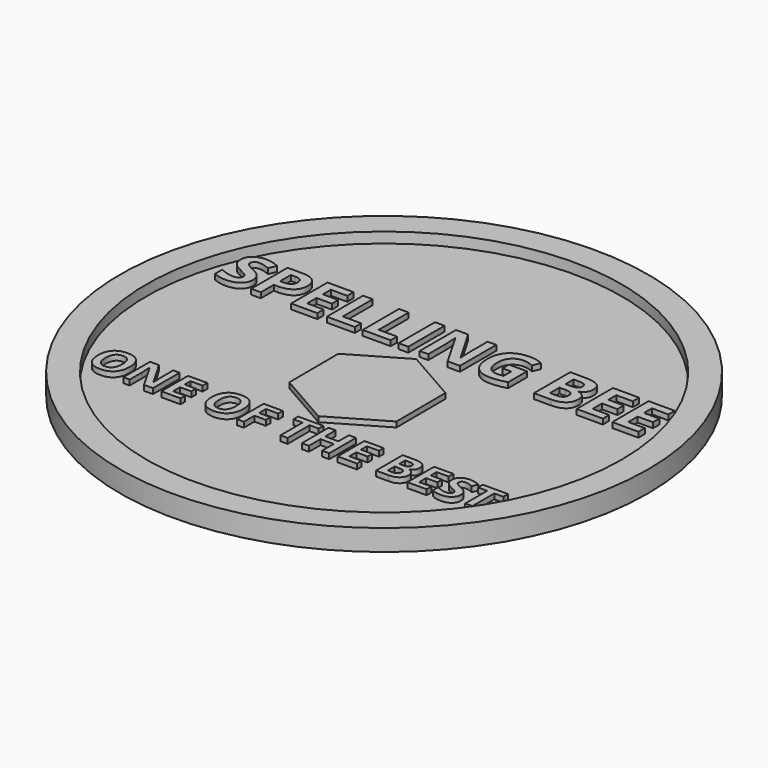
from build123d import *

# Parameters (mm, degrees)
F0_R           = 25
F1_DEPTH       = 1
F2_R           = 25
F2_R_2         = 22.5
F3_DEPTH       = 1
F4_TEXT_SIZE   = 6.0227963006
F4_TEXT_SIZE_2 = 4.4309585139
F5_DEPTH       = 0.5


# Not quite as in the source:
# - Text() gives the source's letters only with a copy of the font that has no kerning and outlines rounded to 1/6400 em; it was checked with that copy


with BuildPart() as f1:
    # F0 (on Top) → F1 (new body)
    with BuildSketch(Plane.XY):
        Circle(F0_R)
    extrude(amount=F1_DEPTH)

    # F2 (on face) → F3 (join)
    with BuildSketch(Plane.XY.offset(1)):
        Circle(F2_R)
        Circle(F2_R_2, mode=Mode.SUBTRACT)
    extrude(amount=F3_DEPTH)

    # F4 (on face) → F5 (join)
    with BuildSketch(Plane.XY.offset(1)):
        Polygon((-0.0296621374, 3.8561042284), (-5.0683934451, 0.9127404655), (-5.0387313077, -4.9226107313), (0.0296621374, -7.8145981652), (5.0683934451, -4.8712344023), (5.0387313077, 0.9641167945), align=None)
        with Locations((-20.4605683074, 5.0238828414)):
            Text('SPELLING BEE', F4_TEXT_SIZE, font='Open Sans', font_style=FontStyle.BOLD, text_align=(TextAlign.LEFT, TextAlign.BOTTOM))
        with Locations((-19.0621219943, -11.9534725112)):
            Text('ONE OF THE BEST', F4_TEXT_SIZE_2, font='Open Sans', font_style=FontStyle.BOLD, text_align=(TextAlign.LEFT, TextAlign.BOTTOM))
    extrude(amount=F5_DEPTH)


solid = f1.part
